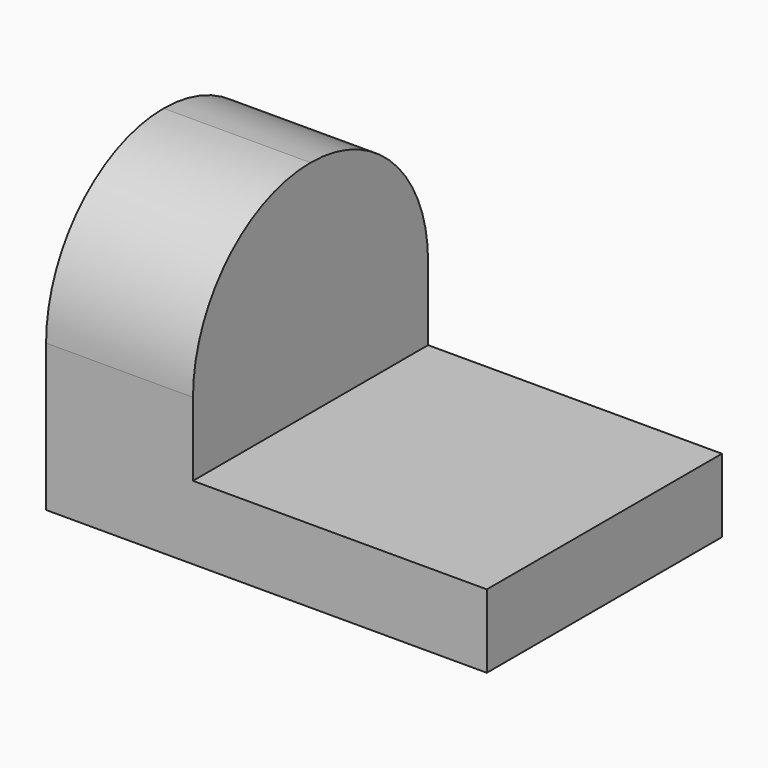
from build123d import *

# Parameters (mm, degrees)
F0_W     = 38.1
F0_H     = 25.4
F1_DEPTH = 25.4
F3_DEPTH = 38.101
F4_DEPTH = 38.101
F5_DEPTH = 25.4


with BuildPart() as f1:
    # F0 (on Top) → F1 (new body)
    with BuildSketch(Plane.XY):
        with Locations((19.05, 12.7)):
            Rectangle(F0_W, F0_H)
    extrude(amount=F1_DEPTH)

    # F2 (on face) → F3 (cut, through all)
    with BuildSketch(Plane.YZ.offset(38.1)):
        with BuildLine():
            ThreePointArc((12.7, 25.4), (21.6802561211, 21.6802561211), (25.4, 12.7))
            Line((25.4, 12.7), (25.4, 25.4))
            Line((25.4, 25.4), (12.7, 25.4))
        make_face()
        with BuildLine():
            ThreePointArc((0, 12.7), (3.7197438789, 21.6802561211), (12.7, 25.4))
            Line((12.7, 25.4), (0, 25.4))
            Line((0, 25.4), (0, 12.7))
        make_face()
    extrude(amount=-F3_DEPTH, mode=Mode.SUBTRACT)

    # F2 (on face) → F4 (cut, through all)
    with BuildSketch(Plane.YZ.offset(38.1)):
        with BuildLine():
            ThreePointArc((12.7, 25.4), (21.6802561211, 21.6802561211), (25.4, 12.7))
            Line((25.4, 12.7), (25.4, 25.4))
            Line((25.4, 25.4), (12.7, 25.4))
        make_face()
    extrude(amount=-F4_DEPTH, mode=Mode.SUBTRACT)

    # F2 (on face) → F5 (cut)
    with BuildSketch(Plane.YZ.offset(38.1)):
        with BuildLine():
            Line((25.4, 6.35), (25.4, 12.7))
            ThreePointArc((25.4, 12.7), (21.6802561211, 21.6802561211), (12.7, 25.4))
            ThreePointArc((12.7, 25.4), (3.7197438789, 21.6802561211), (0, 12.7))
            Line((0, 12.7), (0, 6.35))
            Line((0, 6.35), (25.4, 6.35))
        make_face()
    extrude(amount=-F5_DEPTH, mode=Mode.SUBTRACT)


solid = f1.part
